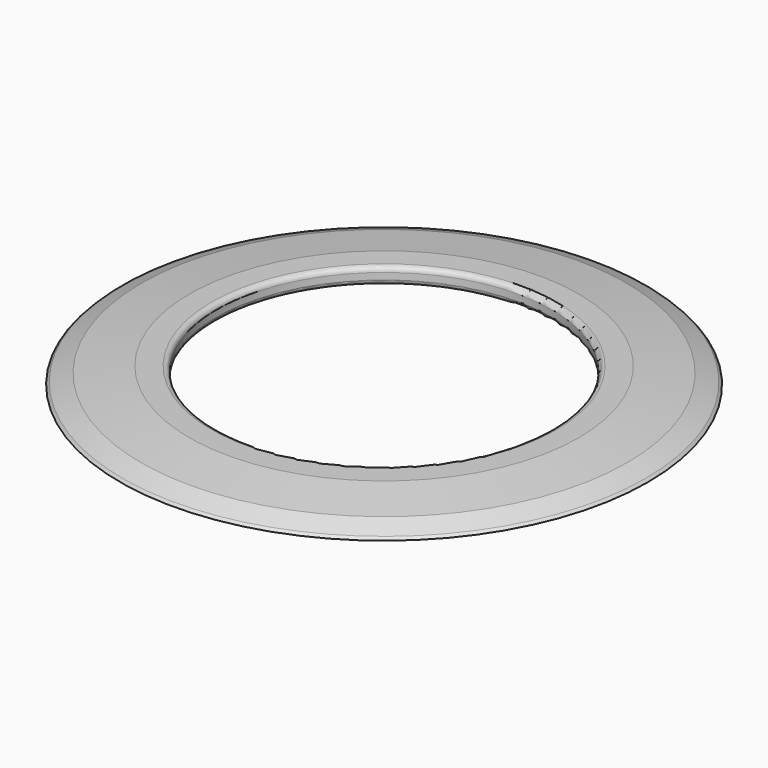
from build123d import *

# Parameters (mm, degrees)
F0_R     = 80
F0_R_2   = 50.8196445325
F1_DEPTH = 5
F2_SIZE  = 4.99999
F3_SIZE  = 6
F4_R     = 1.5
F5_R     = 1.5
F6_SIZE2 = 5
F6_SIZE  = 10


# Not quite as in the source:
# - a fillet or chamfer is up to 0.001 mm smaller than in the source, because OpenCascade refuses the exact size


with BuildPart() as f1:
    # F0 (on Top) → F1 (new body)
    with BuildSketch(Plane.XY):
        Circle(F0_R)
        Circle(F0_R_2, mode=Mode.SUBTRACT)
    extrude(amount=F1_DEPTH)

    # F2 (size 5 in the source; OpenCascade refuses exactly that, so slightly less here)
    f2_edges = [f1.edges().sort_by_distance(p)[0] for p in [
        (-80, 0, 5),
    ]]
    chamfer(f2_edges, length=F2_SIZE)

    # F3
    f3_edges = [f1.edges().sort_by_distance(p)[0] for p in [
        (-75.00001, 0, 5),
    ]]
    chamfer(f3_edges, length=F3_SIZE)

    # F4
    f4_edges = [f1.edges().sort_by_distance(p)[0] for p in [
        (-50.819645, 0, 5),
    ]]
    fillet(f4_edges, radius=F4_R)

    # F5
    f5_edges = [f1.edges().sort_by_distance(p)[0] for p in [
        (-50.819645, 0, 0),
    ]]
    fillet(f5_edges, radius=F5_R)

    # F6
    f6_edges = [f1.edges().sort_by_distance(p)[0] for p in [
        (-69.00001, 0, 5),
    ]]
    chamfer(f6_edges, length=F6_SIZE, length2=F6_SIZE2)


solid = f1.part
